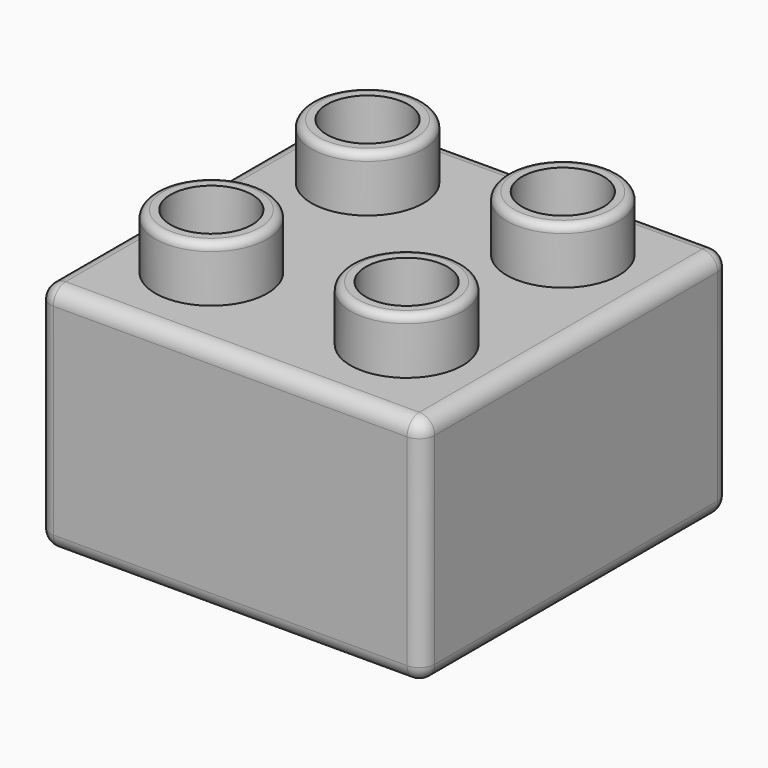
from build123d import *

# Parameters (mm, degrees)
F0_W          = 31.75
F0_H          = 31.75
F5_DEPTH      = 19.177
F1_W          = 28.575
F1_H          = 28.575
F6_DEPTH      = 18.161
F6_DEPTH_BACK = 0.381
F2_R          = 6.5405
F7_DEPTH      = 15.875
F3_R          = 5.461
F8_DEPTH      = 15.875
F8_DEPTH_BACK = 0.635
F4_W          = 1.016
F4_H          = 1.905
F10_DEPTH     = 17.526
F15_ANGLE     = 90
F16_R         = 4.6355
F18_DEPTH     = 4.699
F17_R         = 3.3655
F19_DEPTH     = 4.699
F23_R         = 1.26999
F24_R         = 0.635
F24_2_R       = 0.635
F24_3_R       = 0.635
F24_4_R       = 0.635


# Not quite as in the source:
# - a fillet or chamfer is up to 0.001 mm smaller than in the source, because OpenCascade refuses the exact size


with BuildPart() as f5:
    # F0 (on Top) → F5 (new body)
    with BuildSketch(Plane.XY):
        with Locations((0, -0.3175)):
            Rectangle(F0_W, F0_H)
    extrude(amount=F5_DEPTH)

    # F1 (on face) → F6 (cut, two sides)
    with BuildSketch(Plane.XY) as f6_sk:
        Rectangle(F1_W, F1_H)
    extrude(amount=F6_DEPTH, mode=Mode.SUBTRACT)
    extrude(f6_sk.sketch, amount=-F6_DEPTH_BACK, mode=Mode.SUBTRACT)

    # F23 (radius 1.27 in the source; OpenCascade refuses exactly that, so slightly less here)
    f23_edges = [f5.edges().sort_by_distance(p)[0] for p in [
        (0, -16.1925, 19.177),
        (-15.875, -0.3175, 19.177),
        (0, 15.5575, 19.177),
        (15.875, -0.3175, 19.177),
        (-15.875, -16.1925, 9.5885),
        (15.875, -16.1925, 9.5885),
        (-15.875, 15.5575, 9.5885),
        (15.875, 15.5575, 9.5885),
        (15.875, -0.3175, 0),
        (0, -16.1925, 0),
        (-15.875, -0.3175, 0),
        (0, 15.5575, 0),
    ]]
    fillet(f23_edges, radius=F23_R)


with BuildPart() as f7:
    # F2 (on face) → F7 (new body)
    with BuildSketch(Plane.XY):
        Circle(F2_R)
    extrude(amount=F7_DEPTH)

    # F3 (on face) → F8 (cut, two sides)
    with BuildSketch(Plane.XY) as f8_sk:
        Circle(F3_R)
    extrude(amount=F8_DEPTH, mode=Mode.SUBTRACT)
    extrude(f8_sk.sketch, amount=-F8_DEPTH_BACK, mode=Mode.SUBTRACT)


with BuildPart() as f7_1:
    # F9: moved
    add(f7.part.moved(Location((0, 0, 2.286))))


with BuildPart() as f10:
    # F4 (on face) → F10 (new body)
    with BuildSketch(Plane.XY):
        Rectangle(F4_W, F4_H)
    extrude(amount=F10_DEPTH)


with BuildPart() as f10_1:
    # F11: moved
    add(f10.part.moved(Location((8.0645, 13.8557, 0.635))))


with BuildPart() as f12_1:
    # F12: instance of F10
    add(f10_1.part.mirror(Plane.XZ))


with BuildPart() as f13_1:
    # F13: instance of F12_1
    add(f12_1.part.mirror(Plane.YZ))


with BuildPart() as f13_2:
    # F13: instance of F10
    add(f10_1.part.mirror(Plane.YZ))


with BuildPart() as f15_1:
    # F15: copy of F12_1
    add(f12_1.part.rotate(Axis((0, 0, 4.273429513), (0, 0, -1)), F15_ANGLE))


with BuildPart() as f15_2:
    # F15: copy of F13_1
    add(f13_1.part.rotate(Axis((0, 0, 4.273429513), (0, 0, -1)), F15_ANGLE))


with BuildPart() as f15_3:
    # F15: copy of F10
    add(f10_1.part.rotate(Axis((0, 0, 4.273429513), (0, 0, -1)), F15_ANGLE))


with BuildPart() as f15_4:
    # F15: copy of F13_2
    add(f13_2.part.rotate(Axis((0, 0, 4.273429513), (0, 0, -1)), F15_ANGLE))


with BuildPart() as f18:
    # F16 (on Top) → F18 (new body)
    with BuildSketch(Plane.XY):
        Circle(F16_R)
    extrude(amount=F18_DEPTH)

    # F17 (on Top) → F19 (cut)
    with BuildSketch(Plane.XY):
        Circle(F17_R)
    extrude(amount=F19_DEPTH, mode=Mode.SUBTRACT)


with BuildPart() as f18_1:
    # F20: moved
    add(f18.part.moved(Location((8.0645, 8.0645, 19.05))))


with BuildPart() as f21_1:
    # F21: instance of F18
    add(f18_1.part.mirror(Plane.XZ))


with BuildPart() as f22_1:
    # F22: instance of F18
    add(f18_1.part.mirror(Plane.YZ))

    # F24
    f24_edges = [f22_1.edges().sort_by_distance(p)[0] for p in [
        (-3.429, 8.0645, 23.749),
    ]]
    fillet(f24_edges, radius=F24_R)


with BuildPart() as f22_2:
    # F22: instance of F21_1
    add(f21_1.part.mirror(Plane.YZ))

    # F24#4
    f24_4_edges = [f22_2.edges().sort_by_distance(p)[0] for p in [
        (-3.429, -8.0645, 23.749),
    ]]
    fillet(f24_4_edges, radius=F24_4_R)


with BuildPart() as f18_2:
    add(f18_1.part)

    # F24#2
    f24_2_edges = [f18_2.edges().sort_by_distance(p)[0] for p in [
        (3.429, 8.0645, 23.749),
    ]]
    fillet(f24_2_edges, radius=F24_2_R)


with BuildPart() as f21_1_1:
    add(f21_1.part)

    # F24#3
    f24_3_edges = [f21_1_1.edges().sort_by_distance(p)[0] for p in [
        (3.429, -8.0645, 23.749),
    ]]
    fillet(f24_3_edges, radius=F24_3_R)


solid = Compound([f5.part, f7_1.part, f10_1.part, f12_1.part, f13_1.part, f13_2.part, f15_1.part, f15_2.part, f15_3.part, f15_4.part, f22_1.part, f22_2.part, f18_2.part, f21_1_1.part])
